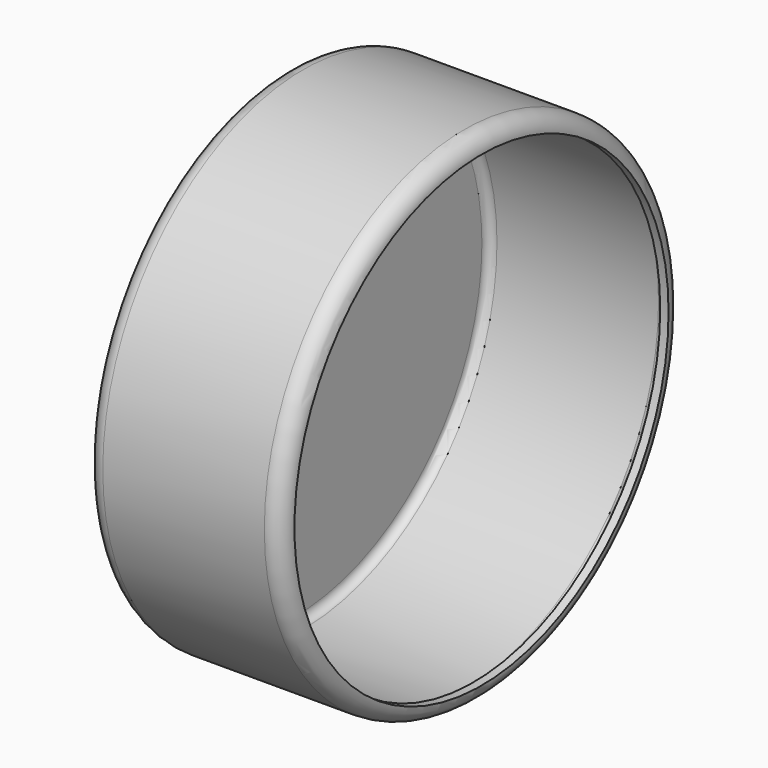
from build123d import *

# Parameters (mm, degrees)
F0_R     = 76.0385345631
F1_DEPTH = 59.182
F2_R     = 5.08
F3_R     = 5.08
F4_T     = -2.54


# Not quite as in the source:
# - a shell that OpenCascade refuses in one call is made with other operations: the cavity is built on its own and cut out


with BuildPart() as f1:
    # F0 (on Right) → F1 (new body)
    with BuildSketch(Plane.YZ):
        Circle(F0_R)
    extrude(amount=F1_DEPTH)

    # F2
    f2_edges = [f1.edges().sort_by_distance(p)[0] for p in [
        (59.182, -76.038535, 0),
    ]]
    fillet(f2_edges, radius=F2_R)

    # F3
    f3_edges = [f1.edges().sort_by_distance(p)[0] for p in [
        (0, -76.038535, 0),
    ]]
    fillet(f3_edges, radius=F3_R)

    # F4: a shell. OpenCascade refuses it in one call, so the cavity is built on its own and cut out:
    # the body offset inwards by the wall thickness, plus a prism from it out through each open face.
    f4_core = offset(f1.part, amount=F4_T, mode=Mode.PRIVATE)
    f4_exits = [f4_core.faces().sort_by_distance(p)[0] for p in [
        (56.642, 0, 0),
    ]]
    add(f4_core, mode=Mode.SUBTRACT)
    extrude(f4_exits, amount=-F4_T, mode=Mode.SUBTRACT)


solid = f1.part
